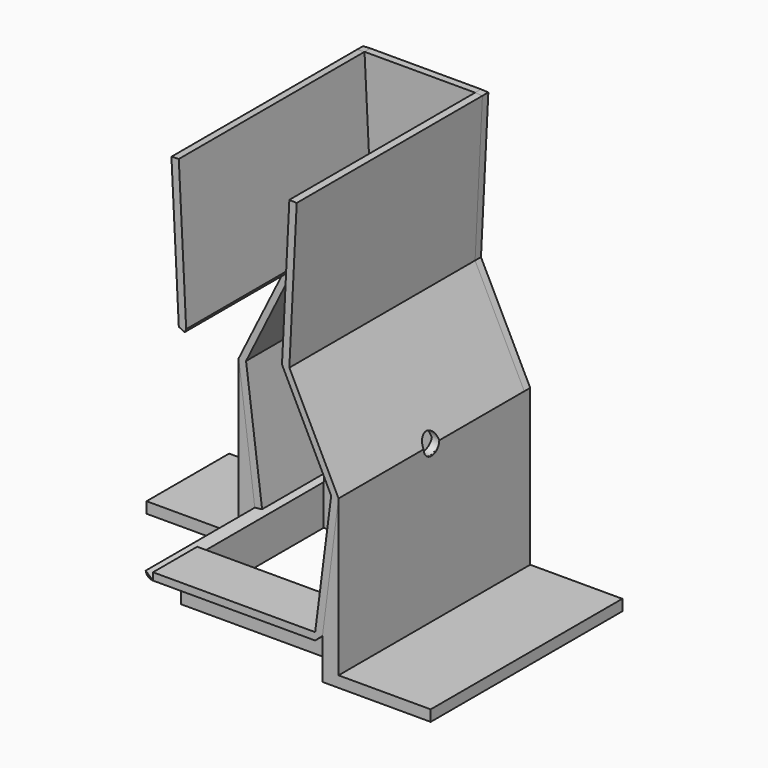
from build123d import *

# Parameters (mm, degrees)
F0_W      = 26
F0_H      = 40
F1_DEPTH  = 2
F3_DEPTH  = 63
F2_W      = 44
F2_H      = 2
F4_DEPTH  = 2
F5_W      = 37
F5_H      = 30.0317472646
F6_DEPTH  = 3
F7_W      = 37
F7_H      = 34.5309597718
F8_DEPTH  = 3
F10_DEPTH = 5
F12_DEPTH = 65
F13_W     = 65
F13_H     = 3
F14_DEPTH = 25
F16_DEPTH = 28
F18_DEPTH = 5
F19_W     = 44
F19_H     = 43
F20_DEPTH = 3
F22_DEPTH = 11


# Not quite as in the source:
# - a feature names something its author has since deleted; it is built from what else it names


with BuildPart() as f1:
    # F0 (on Front) → F1 (new body)
    with BuildSketch(Plane.XZ):
        with Locations((-13, 47)):
            Rectangle(F0_W, F0_H)
        Polygon((-28, 67), (-26, 27), (-26, 67), align=None)
        Polygon((0, 67), (0, 27), (2, 67), align=None)
        with BuildLine():
            Line((-6, 0), (0, 0))
            Line((0, 0), (0, 27))
            Line((0, 27), (-26, 27))
            Line((-26, 27), (-26, 0))
            Line((-26, 0), (-20, 0))
            ThreePointArc((-20, 0), (-13, 7), (-6, 0))
        make_face()
        Polygon((-26, 0), (-26, 27), (-39.35, 0), align=None)
        Polygon((0, 27), (0, 0), (13.35, 0), align=None)
        Polygon((13.35, 0), (0, 0), (0, -34), (9, -34), align=None)
        with BuildLine():
            ThreePointArc((-13, -7), (-17.9497474683, -4.9497474683), (-20, 0))
            Line((-20, 0), (-26, 0))
            Line((-26, 0), (-26, -34))
            Line((-26, -34), (-13, -34))
            Line((-13, -34), (-13, -7))
        make_face()
        Polygon((-26, -34), (-26, 0), (-39.35, 0), (-35, -34), align=None)
        with BuildLine():
            Line((0, -34), (0, 0))
            Line((0, 0), (-6, 0))
            ThreePointArc((-6, 0), (-8.0502525317, -4.9497474683), (-13, -7))
            Line((-13, -7), (-13, -34))
            Line((-13, -34), (0, -34))
        make_face()
    extrude(amount=F1_DEPTH)


with BuildPart() as f3:
    # F2 (on face) → F3 (new body)
    with BuildSketch(Plane.XZ.offset(2)):
        Polygon((-26, 27), (-28, 67), (-29.9975046778, 66.9001247661), (-27.9975046778, 26.9001247661), align=None)
        Polygon((-39.35, 0), (-26, 27), (-27.9975046778, 26.9001247661), (-41.35, 0), align=None)
        Polygon((-35, -34), (-39.35, 0), (-41.35, 0), (-36.9838293096, -34.2538134558), align=None)
    extrude(amount=F3_DEPTH)


with BuildPart() as f3b:
    # F2 (on face) → F3, piece 2 (new body)
    with BuildSketch(Plane.XZ.offset(2)):
        Polygon((3.9975046778, 66.9001247661), (2, 67), (0, 27), (1.9975046778, 26.9001247661), align=None)
        Polygon((1.9975046778, 26.9001247661), (0, 27), (13.35, 0), (15.35, 0), align=None)
        Polygon((15.35, 0), (13.35, 0), (9, -34), (10.9838293096, -34.2538134558), align=None)
        with Locations((-13, -35)):
            Rectangle(F2_W, F2_H)
        Polygon((10.9838293096, -34.2538134558), (9, -34), (9, -36), align=None)
    extrude(amount=F3_DEPTH)


with BuildPart() as f3c:
    # F2 (on face) → F3, piece 3 (new body)
    with BuildSketch(Plane.XZ.offset(2)):
        with BuildLine():
            Line((-35, -36), (-36.9838293096, -34.2538134558))
            ThreePointArc((-36.9838293096, -34.2538134558), (-36.3214335187, -35.5012706138), (-35, -36))
        make_face()
    extrude(amount=F3_DEPTH)


with BuildPart() as f4:
    # F4 (new): a face of the model
    f4_faces = [f3b.part.faces().sort_by_distance(p)[0] for p in [
        (1.8524568997, -2, 46.957377155),
    ]]
    extrude(f4_faces, amount=F4_DEPTH)


with BuildPart() as f4b:
    # F4#2 (new): a face of the model
    f4_2_faces = [f3.part.faces().sort_by_distance(p)[0] for p in [
        (-32.9556846535, -2, 16.3675041089),
    ]]
    extrude(f4_2_faces, amount=F4_DEPTH)


with BuildPart() as f3_1:
    add(f3.part)

    # F5 (on face) → F6 (cut)
    with BuildSketch(Plane(origin=(-33.1759143884, 0, 16.4676277725), x_dir=(0, -1, 0), z_dir=(-0.8957229338, 0, 0.4446126695))):
        with Locations((46.5, -3.3688602532)):
            Rectangle(F5_W, F5_H)
    extrude(amount=-F6_DEPTH, mode=Mode.SUBTRACT)


with BuildPart() as f8_tool:
    # F7 (on face) → F8 (new body)
    with BuildSketch(Plane(origin=(-40.6889114508, 0, -5.1864220266), x_dir=(0, -1, 0), z_dir=(-0.9919739759, 0, -0.1264422049))):
        with Locations((46.5, -12.0370947138)):
            Rectangle(F7_W, F7_H)
    extrude(amount=-F8_DEPTH)


with BuildPart() as f3_2:
    add(f3_1.part)

    # F8: cut by f8_tool
    add(f8_tool.part, mode=Mode.SUBTRACT)


with BuildPart() as f3b_1:
    add(f3b.part)

    # F8: cut by f8_tool
    add(f8_tool.part, mode=Mode.SUBTRACT)

    # F9 (on face) → F10 (cut)
    with BuildSketch(Plane(origin=(15.1045898614, 0, -1.9253102323), x_dir=(0, 1, 0), z_dir=(0.9919739759, 0, -0.1264422049))):
        with BuildLine():
            ThreePointArc((-36.15, 1.940887845), (-33.5, -0.709112155), (-30.85, 1.940887845))
            Line((-30.85, 1.940887845), (-36.15, 1.940887845))
        make_face()
        with BuildLine():
            Line((-36.15, 1.940887845), (-30.85, 1.940887845))
            ThreePointArc((-30.85, 1.940887845), (-33.5, 4.590887845), (-36.15, 1.940887845))
        make_face()
    extrude(amount=-F10_DEPTH, mode=Mode.SUBTRACT)

    # F19 (on face) → F20 (cut)
    with BuildSketch(Plane(origin=(0, 0, -36), x_dir=(1, 0, 0), z_dir=(0, 0, -1))):
        with Locations((-13, 28.5)):
            Rectangle(F19_W, F19_H)
    extrude(amount=-F20_DEPTH, mode=Mode.SUBTRACT)

    # F21 (on face) → F22 (join)
    with BuildSketch(Plane(origin=(0, 0, -36), x_dir=(1, 0, 0), z_dir=(0, 0, -1))):
        Polygon((-35.0963361561, 7), (-35.0963361561, 50.3247156739), (0, 50.3247156739), (0, 7), (2.5343124289, 7), (2.5343124289, 53.2612130046), (-36.8364825845, 53.2612130046), (-36.8364825845, 3.993337974), (-35, 3.993337974), (-35, 7), align=None)
        Polygon((2.5343124289, 7), (0, 7), (-35, 7), (-35, 3.993337974), (2.5343124289, 3.993337974), align=None)
    extrude(amount=F22_DEPTH)


with BuildPart() as f12:
    # F11 (on face) → F12 (new body)
    with BuildSketch(Plane.XZ.offset(65)):
        Polygon((15.35, -45.2538134558), (15.35, 0), (10.9838293096, -34.2538134558), (10.9838293096, -45.2538134558), align=None)
    extrude(amount=-F12_DEPTH)

    # F13 (on face) → F14 (join)
    with BuildSketch(Plane.YZ.offset(15.35)):
        with Locations((-32.5, -43.7538134558)):
            Rectangle(F13_W, F13_H)
    extrude(amount=F14_DEPTH)

    # F17 (on face) → F18 (cut)
    with BuildSketch(Plane.YZ.offset(15.35)):
        with BuildLine():
            Line((-36.1364966571, 0), (-30.8364966571, 0))
            ThreePointArc((-30.8364966571, 0), (-33.4864966571, 2.65), (-36.1364966571, 0))
        make_face()
        with BuildLine():
            ThreePointArc((-36.1364966571, 0), (-33.4864966571, -2.65), (-30.8364966571, 0))
            Line((-30.8364966571, 0), (-36.1364966571, 0))
        make_face()
    extrude(amount=-F18_DEPTH, mode=Mode.SUBTRACT)


with BuildPart() as f16:
    # F15 (on face) → F16 (new body)
    with BuildSketch(Plane(origin=(0, 0, 0), x_dir=(-1, 0, 0), z_dir=(0, 1, 0))):
        Polygon((41.35, -42.2670417726), (41.35, 0), (36.9838293096, -34.2538134558), (36.9838293096, -45.2538134558), (41.35, -45.2538134558), (66.35, -45.2670417726), (66.35, -42.2670417726), align=None)
    extrude(amount=-F16_DEPTH)


solid = Compound([f1.part, f3c.part, f4.part, f4b.part, f3_2.part, f3b_1.part, f12.part, f16.part])
